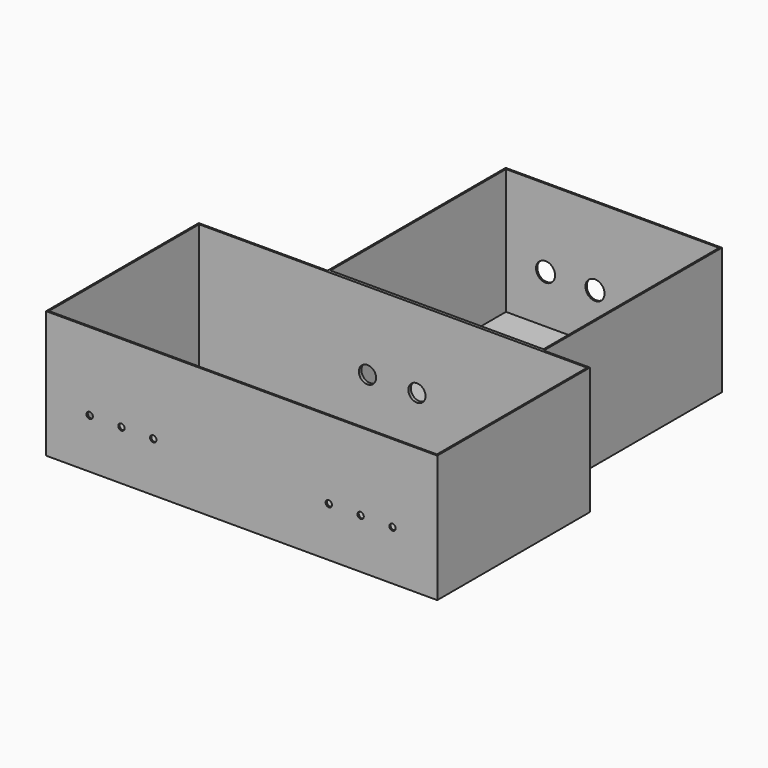
from build123d import *

# Parameters (mm, degrees)
F0_W      = 930
F0_H      = 300
F2_DEPTH  = 200
F3_T      = -2.5
F1_W      = 340
F1_H      = 350
F4_DEPTH  = 200
F5_T      = -2.5
F6_R      = 5
F7_DEPTH  = 25
F8_R      = 13.5
F9_DEPTH  = 25
F10_R     = 15
F11_DEPTH = 25
F12_DEPTH = 160
F13_DEPTH = 160
F14_W     = 300
F14_H     = 200
F15_DEPTH = 2.5
F16_W     = 300
F16_H     = 200
F17_DEPTH = 2.5


# Not quite as in the source:
# - a feature names something its author has since deleted; it is built from what else it names


with BuildPart() as f2:
    # F0 (on Top) → F2 (new body)
    with BuildSketch(Plane.XY):
        Rectangle(F0_W, F0_H)
    extrude(amount=F2_DEPTH)

    # F3
    f3_openings = [f2.faces().sort_by_distance(p)[0] for p in [
        (0, 0, 200),
    ]]
    offset(amount=F3_T, openings=f3_openings)

    # F6 (on face) → F7 (cut)
    with BuildSketch(Plane.XZ.offset(150)):
        with Locations((137, 78.065)):
            Circle(F6_R)
        with Locations((187, 78.065)):
            Circle(F6_R)
        with Locations((237, 78.065)):
            Circle(F6_R)
        with Locations((387, 78.065)):
            Circle(F6_R)
        with Locations((337, 78.065)):
            Circle(F6_R)
        with Locations((-139, 78.065)):
            Circle(F6_R)
        with Locations((-189, 78.065)):
            Circle(F6_R)
        with Locations((-239, 78.065)):
            Circle(F6_R)
        with Locations((-339, 78.065)):
            Circle(F6_R)
        with Locations((-389, 78.065)):
            Circle(F6_R)
    extrude(amount=-F7_DEPTH, mode=Mode.SUBTRACT)


with BuildPart() as f4:
    # F1 (on Top) → F4 (new body)
    with BuildSketch(Plane.XY):
        with Locations((65, 325)):
            Rectangle(F1_W, F1_H)
    extrude(amount=F4_DEPTH)

    # F5
    f5_openings = [f4.faces().sort_by_distance(p)[0] for p in [
        (65, 325, 200),
    ]]
    offset(amount=F5_T, openings=f5_openings)


with BuildPart() as f9_tool:
    # F8 (on face) → F9 (new body)
    with BuildSketch(Plane.XZ.offset(-147.5)):
        with Locations((37.505, 78.065)):
            Circle(F8_R)
        with Locations((-40.25, 78.065)):
            Circle(F8_R)
    extrude(amount=-F9_DEPTH)


with BuildPart() as f2_1:
    add(f2.part)

    # F9: cut by f9_tool
    add(f9_tool.part, mode=Mode.SUBTRACT)

    # F12 (cut): a face of the model
    f12_faces = [f2_1.faces().sort_by_distance(p)[0] for p in [
        (-465, 0, 100),
    ]]
    extrude(f12_faces, amount=-F12_DEPTH, mode=Mode.SUBTRACT)

    # F13 (cut): a face of the model
    f13_faces = [f2_1.faces().sort_by_distance(p)[0] for p in [
        (465, 0, 100),
    ]]
    extrude(f13_faces, amount=-F13_DEPTH, mode=Mode.SUBTRACT)

    # F14 (on face) → F15 (join)
    with BuildSketch(Plane.YZ.offset(305)):
        with Locations((0, 100)):
            Rectangle(F14_W, F14_H)
    extrude(amount=F15_DEPTH)

    # F16 (on face) → F17 (join)
    with BuildSketch(Plane(origin=(-305, 0, 0), x_dir=(0, -1, 0), z_dir=(-1, 0, 0))):
        with Locations((0, 100)):
            Rectangle(F16_W, F16_H)
    extrude(amount=F17_DEPTH)


with BuildPart() as f4_1:
    add(f4.part)

    # F9: cut by f9_tool
    add(f9_tool.part, mode=Mode.SUBTRACT)

    # F10 (on face) → F11 (cut)
    with BuildSketch(Plane(origin=(0, 500, 0), x_dir=(-1, 0, 0), z_dir=(0, 1, 0))):
        with Locations((-37.505, 78.065)):
            Circle(F10_R)
        with Locations((40.25, 78.065)):
            Circle(F10_R)
    extrude(amount=-F11_DEPTH, mode=Mode.SUBTRACT)


solid = Compound([f2_1.part, f4_1.part])
